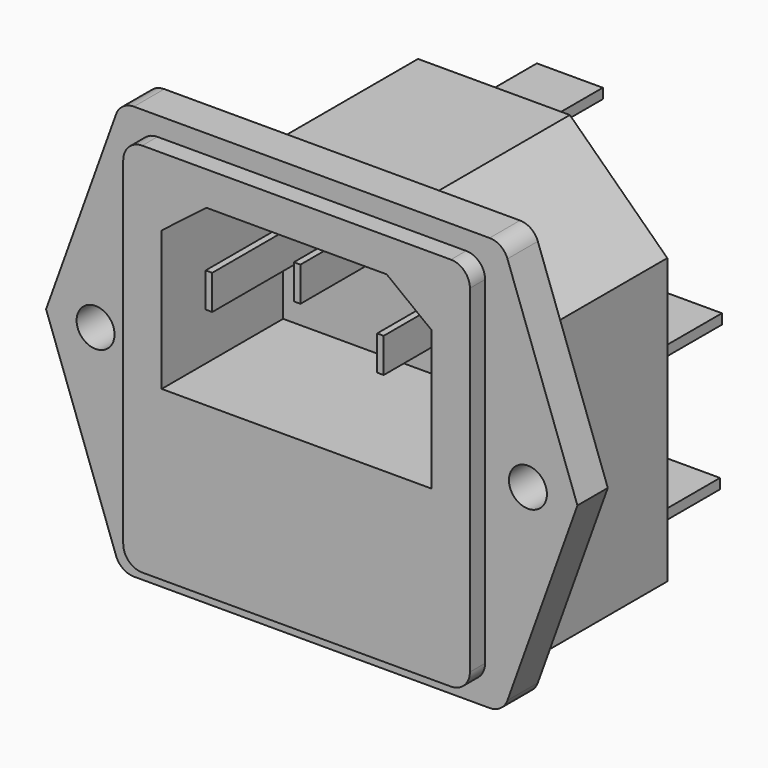
from build123d import *

# Parameters (mm, degrees)
F0_R     = 1.5875
F1_DEPTH = 3.175
F3_DEPTH = 1.5875
F5_DEPTH = 15.875
F6_W     = 5.5154263973
F6_H     = 0.8426345885
F7_DEPTH = 7.9375
F8_W     = 0.5498970859
F8_H     = 2.8869584203
F9_DEPTH = 12.7


# Not quite as in the source:
# - a feature names something its author has since deleted; it is built from what else it names


with BuildPart() as f1:
    # F0 (on Front) → F1 (new body)
    with BuildSketch(Plane.XZ):
        with BuildLine():
            ThreePointArc((16.3714576415, 16.2581077061), (15.790628657, 17.019159057), (14.8778171338, 17.3078398343))
            Line((14.8778171338, 17.3078398343), (-14.8778171338, 17.3078398343))
            ThreePointArc((-14.8778171338, 17.3078398343), (-15.790628657, 17.019159057), (-16.3714576415, 16.2581077061))
            Line((-16.3714576415, 16.2581077061), (-22.225, 0))
            Line((-22.225, 0), (-16.3714576415, -16.2581077061))
            ThreePointArc((-16.3714576415, -16.2581077061), (-15.790628657, -17.019159057), (-14.8778171338, -17.3078398343))
            Line((-14.8778171338, -17.3078398343), (14.8778171338, -17.3078398343))
            ThreePointArc((14.8778171338, -17.3078398343), (15.790628657, -17.019159057), (16.3714576415, -16.2581077061))
            Line((16.3714576415, -16.2581077061), (22.225, 0))
            Line((22.225, 0), (16.3714576415, 16.2581077061))
        make_face()
        with Locations((-18.0848, 0)):
            Circle(F0_R, mode=Mode.SUBTRACT)
        with BuildLine():
            ThreePointArc((-14.4999964, 14.1328398343), (-14.0350284151, 15.2553718495), (-12.9124964, 15.7203398343))
            Line((-12.9124964, 15.7203398343), (12.9124964, 15.7203398343))
            ThreePointArc((12.9124964, 15.7203398343), (14.0350284151, 15.2553718495), (14.4999964, 14.1328398343))
            Line((14.4999964, 14.1328398343), (14.4999964, -14.1328398343))
            ThreePointArc((14.4999964, -14.1328398343), (14.0350284151, -15.2553718495), (12.9124964, -15.7203398343))
            Line((12.9124964, -15.7203398343), (-12.9124964, -15.7203398343))
            ThreePointArc((-12.9124964, -15.7203398343), (-14.0350284151, -15.2553718495), (-14.4999964, -14.1328398343))
            Line((-14.4999964, -14.1328398343), (-14.4999964, 14.1328398343))
        make_face(mode=Mode.SUBTRACT)
        with Locations((18.0848, 0)):
            Circle(F0_R, mode=Mode.SUBTRACT)
        with BuildLine():
            Line((12.9124964, 15.7203398343), (-12.9124964, 15.7203398343))
            ThreePointArc((-12.9124964, 15.7203398343), (-14.0350284151, 15.2553718495), (-14.4999964, 14.1328398343))
            Line((-14.4999964, 14.1328398343), (-14.4999964, -14.1328398343))
            ThreePointArc((-14.4999964, -14.1328398343), (-14.0350284151, -15.2553718495), (-12.9124964, -15.7203398343))
            Line((-12.9124964, -15.7203398343), (12.9124964, -15.7203398343))
            ThreePointArc((12.9124964, -15.7203398343), (14.0350284151, -15.2553718495), (14.4999964, -14.1328398343))
            Line((14.4999964, -14.1328398343), (14.4999964, 14.1328398343))
            ThreePointArc((14.4999964, 14.1328398343), (14.0350284151, 15.2553718495), (12.9124964, 15.7203398343))
        make_face()
    extrude(amount=F1_DEPTH)

    # F2 (on face) → F3 (join)
    with BuildSketch(Plane.XZ.offset(3.175)):
        with BuildLine():
            Line((12.9124964, 15.7203398343), (-12.9124964, 15.7203398343))
            ThreePointArc((-12.9124964, 15.7203398343), (-14.0350284151, 15.2553718495), (-14.4999964, 14.1328398343))
            Line((-14.4999964, 14.1328398343), (-14.4999964, -14.1328398343))
            ThreePointArc((-14.4999964, -14.1328398343), (-14.0350284151, -15.2553718495), (-12.9124964, -15.7203398343))
            Line((-12.9124964, -15.7203398343), (12.9124964, -15.7203398343))
            ThreePointArc((12.9124964, -15.7203398343), (14.0350284151, -15.2553718495), (14.4999964, -14.1328398343))
            Line((14.4999964, -14.1328398343), (14.4999964, 14.1328398343))
            ThreePointArc((14.4999964, 14.1328398343), (14.0350284151, 15.2553718495), (12.9124964, 15.7203398343))
        make_face()
    extrude(amount=F3_DEPTH)

    # F4 (on face) → F5 (join)
    with BuildSketch(Plane(origin=(0, 0, 0), x_dir=(-1, 0, 0), z_dir=(0, 1, 0))):
        Polygon((6.35, 15.8496), (-6.35, 15.8496), (-14.5034, 7.9629), (-14.5034, -15.8496), (14.5034, -15.8496), (14.5034, 7.9629), align=None)
    extrude(amount=F5_DEPTH)

    # F6 (on face) → F7 (join)
    with BuildSketch(Plane(origin=(0, 15.875, 0), x_dir=(-1, 0, 0), z_dir=(0, 1, 0))):
        with Locations((0.0007232884, 13.041603379)):
            Rectangle(F6_W, F6_H)
        with Locations((-9.964916273, -0.3249486908)):
            Rectangle(F6_W, F6_H)
        with Locations((-9.8044754704, -12.5053403899)):
            Rectangle(F6_W, F6_H)
    extrude(amount=F7_DEPTH)

    # F8 (on face) → F9 (cut)
    with BuildSketch(Plane.XZ.offset(4.7625)):
        Polygon((-11.2841911614, 10.0093806594), (-11.2841911614, -1.6703880579), (11.2841911614, -1.6703880579), (11.2841911614, 10.0093806594), (7.5404811705, 12.8898254096), (-7.5404811705, 12.8898254096), align=None)
        with Locations((-7.3291899171, 6.8128034472)):
            Rectangle(F8_W, F8_H, mode=Mode.SUBTRACT)
        with Locations((7.0140829775, 6.8357163109)):
            Rectangle(F8_W, F8_H, mode=Mode.SUBTRACT)
        with Locations((0.0484438497, 9.8143247887)):
            Rectangle(F8_W, F8_H, mode=Mode.SUBTRACT)
    extrude(amount=-F9_DEPTH, mode=Mode.SUBTRACT)


solid = f1.part
